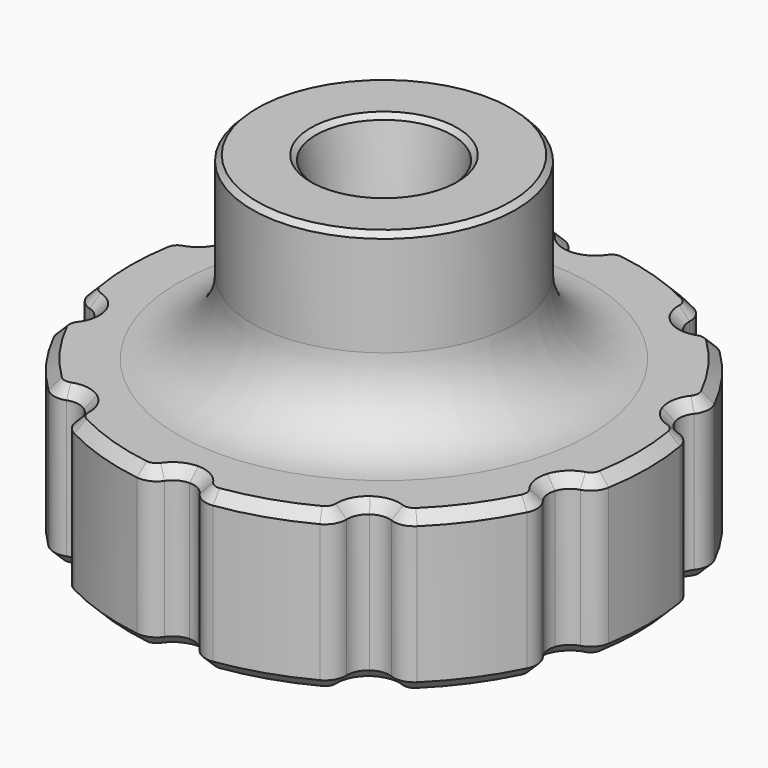
from build123d import *

# Parameters (mm, degrees)
F0_R            = 25
F1_DEPTH        = 15
F3_DEPTH        = 25
F4_R            = 12.5
F5_DEPTH        = 17
F10_D           = 5.5
F10_CBORE_D     = 9
F10_CBORE_DEPTH = 7
F11_R           = 7
F13_SIZE        = 1


# Not quite as in the source:
# - a fillet or chamfer that OpenCascade refuses, or shapes differently, is made with other operations: its cross-section is extruded or revolved along the edge and cut away or added


with BuildPart() as f1:
    # F0 (on Top) → F1 (new body)
    with BuildSketch(Plane.XY):
        Circle(F0_R)
    extrude(amount=F1_DEPTH)

    # F2 (on face) → F3 (cut)
    with BuildSketch(Plane(origin=(0, 0, 0), x_dir=(1, 0, 0), z_dir=(0, 0, -1))):
        with BuildLine():
            ThreePointArc((-12.695782627, 20.2932772978), (-12.4260089018, 21.3662664433), (-11.6271021161, 22.1316627568))
            ThreePointArc((-11.6271021161, 22.1316627568), (-14.6946313073, 20.2254248594), (-17.4554899321, 17.8970911388))
            ThreePointArc((-17.4554899321, 17.8970911388), (-16.4806790069, 18.420376175), (-15.3768410224, 18.3453743535))
            ThreePointArc((-15.3768410224, 18.3453743535), (-14.4153207616, 18.245024491), (-13.5190608027, 18.6073908706))
            ThreePointArc((-13.5190608027, 18.6073908706), (-12.8974703374, 19.3478073753), (-12.695782627, 20.2932772978))
        make_face()
        with BuildLine():
            ThreePointArc((-1.6569852142, 23.88), (-0.938083152, 23.2336478267), (0, 23))
            ThreePointArc((0, 23), (0.938083152, 23.2336478267), (1.6569852142, 23.88))
            ThreePointArc((1.6569852142, 23.88), (2.5059239381, 24.5894974363), (3.6021417699, 24.7391304348))
            ThreePointArc((3.6021417699, 24.7391304348), (0, 25), (-3.6021417699, 24.7391304348))
            ThreePointArc((-3.6021417699, 24.7391304348), (-2.5059239381, 24.5894974363), (-1.6569852142, 23.88))
        make_face()
        with BuildLine():
            ThreePointArc((17.4554899321, 17.8970911388), (14.6946313073, 20.2254248594), (11.6271021161, 22.1316627568))
            ThreePointArc((11.6271021161, 22.1316627568), (12.4260089018, 21.3662664433), (12.695782627, 20.2932772978))
            ThreePointArc((12.695782627, 20.2932772978), (12.8974703374, 19.3478073753), (13.5190608027, 18.6073908706))
            ThreePointArc((13.5190608027, 18.6073908706), (14.4153207616, 18.245024491), (15.3768410224, 18.3453743535))
            ThreePointArc((15.3768410224, 18.3453743535), (16.4806790069, 18.420376175), (17.4554899321, 17.8970911388))
        make_face()
        with BuildLine():
            ThreePointArc((24.6414342305, 4.2189713275), (23.7764129074, 7.7254248594), (22.4151881844, 11.0706521333))
            ThreePointArc((22.4151881844, 11.0706521333), (22.6116286858, 9.9818478816), (22.1991930185, 8.955212411))
            ThreePointArc((22.1991930185, 8.955212411), (21.8066285268, 8.0717621143), (21.8742998748, 7.1073908706))
            ThreePointArc((21.8742998748, 7.1073908706), (22.386395799, 6.2874219253), (23.2232661997, 5.8034392403))
            ThreePointArc((23.2232661997, 5.8034392403), (24.1603748527, 5.2152973003), (24.6414342305, 4.2189713275))
        make_face()
        with BuildLine():
            ThreePointArc((22.4151881844, -11.0706521333), (23.7764129074, -7.7254248594), (24.6414342305, -4.2189713275))
            ThreePointArc((24.6414342305, -4.2189713275), (24.1603748527, -5.2152973003), (23.2232661997, -5.8034392403))
            ThreePointArc((23.2232661997, -5.8034392403), (22.386395799, -6.2874219253), (21.8742998748, -7.1073908706))
            ThreePointArc((21.8742998748, -7.1073908706), (21.8066285268, -8.0717621143), (22.1991930185, -8.955212411))
            ThreePointArc((22.1991930185, -8.955212411), (22.6116286858, -9.9818478816), (22.4151881844, -11.0706521333))
        make_face()
        with BuildLine():
            ThreePointArc((11.6271021161, -22.1316627568), (14.6946313073, -20.2254248594), (17.4554899321, -17.8970911388))
            ThreePointArc((17.4554899321, -17.8970911388), (16.4806790069, -18.420376175), (15.3768410224, -18.3453743535))
            ThreePointArc((15.3768410224, -18.3453743535), (14.4153207616, -18.245024491), (13.5190608027, -18.6073908706))
            ThreePointArc((13.5190608027, -18.6073908706), (12.8974703374, -19.3478073753), (12.695782627, -20.2932772978))
            ThreePointArc((12.695782627, -20.2932772978), (12.4260089018, -21.3662664433), (11.6271021161, -22.1316627568))
        make_face()
        with BuildLine():
            ThreePointArc((-1.6569852142, -23.88), (-2.5059239381, -24.5894974363), (-3.6021417699, -24.7391304348))
            ThreePointArc((-3.6021417699, -24.7391304348), (0, -25), (3.6021417699, -24.7391304348))
            ThreePointArc((3.6021417699, -24.7391304348), (2.5059239381, -24.5894974363), (1.6569852142, -23.88))
            ThreePointArc((1.6569852142, -23.88), (0.938083152, -23.2336478267), (0, -23))
            ThreePointArc((0, -23), (-0.938083152, -23.2336478267), (-1.6569852142, -23.88))
        make_face()
        with BuildLine():
            ThreePointArc((-15.3768410224, -18.3453743535), (-16.4806790069, -18.420376175), (-17.4554899321, -17.8970911388))
            ThreePointArc((-17.4554899321, -17.8970911388), (-14.6946313073, -20.2254248594), (-11.6271021161, -22.1316627568))
            ThreePointArc((-11.6271021161, -22.1316627568), (-12.4260089018, -21.3662664433), (-12.695782627, -20.2932772978))
            ThreePointArc((-12.695782627, -20.2932772978), (-12.8974703374, -19.3478073753), (-13.5190608027, -18.6073908706))
            ThreePointArc((-13.5190608027, -18.6073908706), (-14.4153207616, -18.245024491), (-15.3768410224, -18.3453743535))
        make_face()
        with BuildLine():
            ThreePointArc((-23.2232661997, -5.8034392403), (-24.1603748527, -5.2152973003), (-24.6414342305, -4.2189713275))
            ThreePointArc((-24.6414342305, -4.2189713275), (-23.7764129074, -7.7254248594), (-22.4151881844, -11.0706521333))
            ThreePointArc((-22.4151881844, -11.0706521333), (-22.6116286858, -9.9818478816), (-22.1991930185, -8.955212411))
            ThreePointArc((-22.1991930185, -8.955212411), (-21.8066285268, -8.0717621143), (-21.8742998748, -7.1073908706))
            ThreePointArc((-21.8742998748, -7.1073908706), (-22.386395799, -6.2874219253), (-23.2232661997, -5.8034392403))
        make_face()
        with BuildLine():
            ThreePointArc((-22.1991930185, 8.955212411), (-22.6116286858, 9.9818478816), (-22.4151881844, 11.0706521333))
            ThreePointArc((-22.4151881844, 11.0706521333), (-23.7764129074, 7.7254248594), (-24.6414342305, 4.2189713275))
            ThreePointArc((-24.6414342305, 4.2189713275), (-24.1603748527, 5.2152973003), (-23.2232661997, 5.8034392403))
            ThreePointArc((-23.2232661997, 5.8034392403), (-22.386395799, 6.2874219253), (-21.8742998748, 7.1073908706))
            ThreePointArc((-21.8742998748, 7.1073908706), (-21.8066285268, 8.0717621143), (-22.1991930185, 8.955212411))
        make_face()
    extrude(amount=-F3_DEPTH, mode=Mode.SUBTRACT)

    # F4 (on face) → F5 (join)
    with BuildSketch(Plane.XY.offset(15)):
        Circle(F4_R)
    extrude(amount=F5_DEPTH)

    # F7 (on Right) → F8 (revolve, cut)
    with BuildSketch(Plane.YZ):
        Polygon((6.5, 32), (0, 32), (0, 12), (5, 12), (5, 21), align=None)
    revolve(axis=Axis((0, 0, 22), (0, 0, -1)), mode=Mode.SUBTRACT)

    # F10 (through all)
    with Locations(Plane(origin=(0, 0, 0), x_dir=(1, 0, 0), z_dir=(0, 0, -1))):
        with Locations((0, 0)):
            CounterBoreHole(F10_D / 2, F10_CBORE_D / 2, F10_CBORE_DEPTH)

    # F11
    f11_edges = [f1.edges().sort_by_distance(p)[0] for p in [
        (-12.5, 0, 15),
    ]]
    fillet(f11_edges, radius=F11_R)

    # F12: chamfer of 0.5 on 3 edges, made by hand

    # F12_s1 → F12_t2 (revolve, cut)
    with BuildSketch(Plane.XZ):
        Polygon((12.5, 31.5), (12, 32), (12.5, 32), align=None)
    revolve(axis=Axis((0, 0, 32), (0, 0, 1)), mode=Mode.SUBTRACT)

    # F12_s3 → F12_t4 (revolve, cut)
    with BuildSketch(Plane.YZ):
        Polygon((6.9364455298, 32), (6.4410304458, 31.5675566024), (6.5, 32), align=None)
    revolve(axis=Axis((0, 0, 32), (0, 0, -1)), mode=Mode.SUBTRACT)

    # F12_s5 → F12_t6 (revolve, cut)
    with BuildSketch(Plane.XZ):
        Polygon((5, 0), (4.5, 0.5), (4.5, 0), align=None)
    revolve(axis=Axis((0, 0, 0), (0, 0, -1)), mode=Mode.SUBTRACT)

    # F13
    f13_edges = [f1.edges().sort_by_distance(p)[0] for p in [
        (-25, 0, 0),
        (-25, 0, 15),
        (24.160375, -5.215297, 15),
        (25, 0, 15),
        (21.8743, -7.107391, 15),
        (24.160375, 5.215297, 15),
        (22.611629, -9.981848, 15),
        (21.8743, 7.107391, 15),
        (20.225425, -14.694631, 15),
        (22.611629, 9.981848, 15),
        (16.480679, -18.420376, 15),
        (20.225425, 14.694631, 15),
        (13.519061, -18.607391, 15),
        (16.480679, 18.420376, 15),
        (12.426009, -21.366266, 15),
        (13.519061, 18.607391, 15),
        (7.725425, -23.776413, 15),
        (12.426009, 21.366266, 15),
        (2.505924, -24.589497, 15),
        (7.725425, 23.776413, 15),
        (0, -23, 15),
        (2.505924, 24.589497, 15),
        (-2.505924, -24.589497, 15),
        (0, 23, 15),
        (-7.725425, -23.776413, 15),
        (-2.505924, 24.589497, 15),
        (-12.426009, -21.366266, 15),
        (-7.725425, 23.776413, 15),
        (-13.519061, -18.607391, 15),
        (-12.426009, 21.366266, 15),
        (-16.480679, -18.420376, 15),
        (-13.519061, 18.607391, 15),
        (-20.225425, -14.694631, 15),
        (-16.480679, 18.420376, 15),
        (-22.611629, -9.981848, 15),
        (-20.225425, 14.694631, 15),
        (-21.8743, -7.107391, 15),
        (-22.611629, 9.981848, 15),
        (-24.160375, -5.215297, 15),
        (-21.8743, 7.107391, 15),
        (-24.160375, 5.215297, 15),
        (24.160375, -5.215297, 0),
        (25, 0, 0),
        (21.8743, -7.107391, 0),
        (24.160375, 5.215297, 0),
        (22.611629, -9.981848, 0),
        (21.8743, 7.107391, 0),
        (20.225425, -14.694631, 0),
        (22.611629, 9.981848, 0),
        (16.480679, -18.420376, 0),
        (20.225425, 14.694631, 0),
        (13.519061, -18.607391, 0),
        (16.480679, 18.420376, 0),
        (12.426009, -21.366266, 0),
        (13.519061, 18.607391, 0),
        (7.725425, -23.776413, 0),
        (12.426009, 21.366266, 0),
        (2.505924, -24.589497, 0),
        (7.725425, 23.776413, 0),
        (0, -23, 0),
        (2.505924, 24.589497, 0),
        (-2.505924, -24.589497, 0),
        (0, 23, 0),
        (-7.725425, -23.776413, 0),
        (-2.505924, 24.589497, 0),
        (-12.426009, -21.366266, 0),
        (-7.725425, 23.776413, 0),
        (-13.519061, -18.607391, 0),
        (-12.426009, 21.366266, 0),
        (-16.480679, -18.420376, 0),
        (-13.519061, 18.607391, 0),
        (-20.225425, -14.694631, 0),
        (-16.480679, 18.420376, 0),
        (-22.611629, -9.981848, 0),
        (-20.225425, 14.694631, 0),
        (-21.8743, -7.107391, 0),
        (-22.611629, 9.981848, 0),
        (-24.160375, -5.215297, 0),
        (-21.8743, 7.107391, 0),
        (-24.160375, 5.215297, 0),
    ]]
    chamfer(f13_edges, length=F13_SIZE)


solid = f1.part
